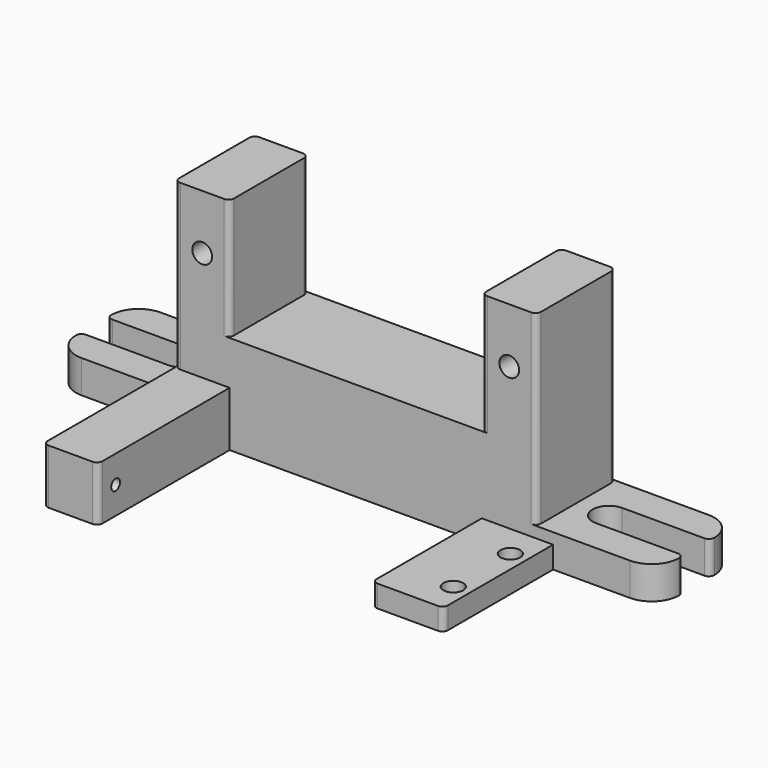
from build123d import *

# Parameters (mm, degrees)
F0_W      = 5
F0_H      = 9
F0_W_2    = 23
F1_DEPTH  = 3
F2_DEPTH  = 20
F3_DEPTH  = 9
F0_H_2    = 15
F4_DEPTH  = 5
F5_R      = 0.5
F6_DEPTH  = 25
F7_W      = 6.5
F7_H      = 12.5
F7_R      = 0.9
F8_DEPTH  = 2
F9_R      = 0.9
F10_DEPTH = 25
F11_R     = 0.49999


# Not quite as in the source:
# - a fillet or chamfer is up to 0.001 mm smaller than in the source, because OpenCascade refuses the exact size


with BuildPart() as f1:
    # F0 (on Top) → F1 (new body)
    with BuildSketch(Plane.XY):
        with BuildLine():
            Line((-16.5, 4.5), (-25, 4.5))
            ThreePointArc((-25, 4.5), (-26.767766953, 3.767766953), (-27.5, 2))
            Line((-27.5, 2), (-27.5, 1.5))
            Line((-27.5, 1.5), (-19.5, 1.5))
            ThreePointArc((-19.5, 1.5), (-18, 0), (-19.5, -1.5))
            Line((-19.5, -1.5), (-27.5, -1.5))
            Line((-27.5, -1.5), (-27.5, -2))
            ThreePointArc((-27.5, -2), (-26.767766953, -3.767766953), (-25, -4.5))
            Line((-25, -4.5), (-16.5, -4.5))
            Line((-16.5, -4.5), (-16.5, 4.5))
        make_face()
        with BuildLine():
            Line((25, 4.5), (16.5, 4.5))
            Line((16.5, 4.5), (16.5, -4.5))
            Line((16.5, -4.5), (25, -4.5))
            ThreePointArc((25, -4.5), (26.767766953, -3.767766953), (27.5, -2))
            Line((27.5, -2), (27.5, -1.5))
            Line((27.5, -1.5), (19.5, -1.5))
            ThreePointArc((19.5, -1.5), (18, 0), (19.5, 1.5))
            Line((19.5, 1.5), (27.5, 1.5))
            Line((27.5, 1.5), (27.5, 2))
            ThreePointArc((27.5, 2), (26.767766953, 3.767766953), (25, 4.5))
        make_face()
        with Locations((-14, 0)):
            Rectangle(F0_W, F0_H)
        with Locations((14, 0)):
            Rectangle(F0_W, F0_H)
        Rectangle(F0_W_2, F0_H)
    extrude(amount=F1_DEPTH)

    # F0 (on Top) → F2 (join)
    with BuildSketch(Plane.XY):
        with Locations((14, 0)):
            Rectangle(F0_W, F0_H)
        with Locations((-14, 0)):
            Rectangle(F0_W, F0_H)
    extrude(amount=F2_DEPTH)

    # F0 (on Top) → F3 (join)
    with BuildSketch(Plane.XY):
        Rectangle(F0_W_2, F0_H)
    extrude(amount=F3_DEPTH)

    # F0 (on Top) → F4 (join)
    with BuildSketch(Plane.XY):
        with Locations((-14, -12)):
            Rectangle(F0_W, F0_H_2)
    extrude(amount=F4_DEPTH)

    # F5 (on face) → F6 (cut)
    with BuildSketch(Plane.YZ.offset(-11.5)):
        with Locations((-17.5, 2.5)):
            Circle(F5_R)
    extrude(amount=-F6_DEPTH, mode=Mode.SUBTRACT)

    # F7 (on Top) → F8 (join)
    with BuildSketch(Plane.XY):
        with Locations((14.75, -10.75)):
            Rectangle(F7_W, F7_H)
        with Locations((16.5, -14)):
            Circle(F7_R, mode=Mode.SUBTRACT)
        with Locations((16.5, -7.5)):
            Circle(F7_R, mode=Mode.SUBTRACT)
    extrude(amount=F8_DEPTH)

    # F9 (on face) → F10 (cut)
    with BuildSketch(Plane.XZ.offset(4.5)):
        with Locations((-14, 15)):
            Circle(F9_R)
        with Locations((14, 15)):
            Circle(F9_R)
    extrude(amount=-F10_DEPTH, mode=Mode.SUBTRACT)

    # F11 (radius 0.5 in the source; OpenCascade refuses exactly that, so slightly less here)
    f11_edges = [f1.edges().sort_by_distance(p)[0] for p in [
        (11.5, -17, 1),
        (18, -17, 1),
        (-11.5, -19.5, 2.5),
        (-16.5, -19.5, 2.5),
        (-16.5, -4.5, 12.5),
        (11.5, -4.5, 14.5),
        (-11.5, -4.5, 14.5),
        (16.5, -4.5, 11.5),
        (11.5, 4.5, 14.5),
        (-11.5, 4.5, 14.5),
        (-16.5, 4.5, 11.5),
        (16.5, 4.5, 11.5),
        (-27.5, 1.5, 1.5),
        (-27.5, -1.5, 1.5),
        (27.5, 1.5, 1.5),
        (27.5, -1.5, 1.5),
    ]]
    fillet(f11_edges, radius=F11_R)


solid = f1.part
